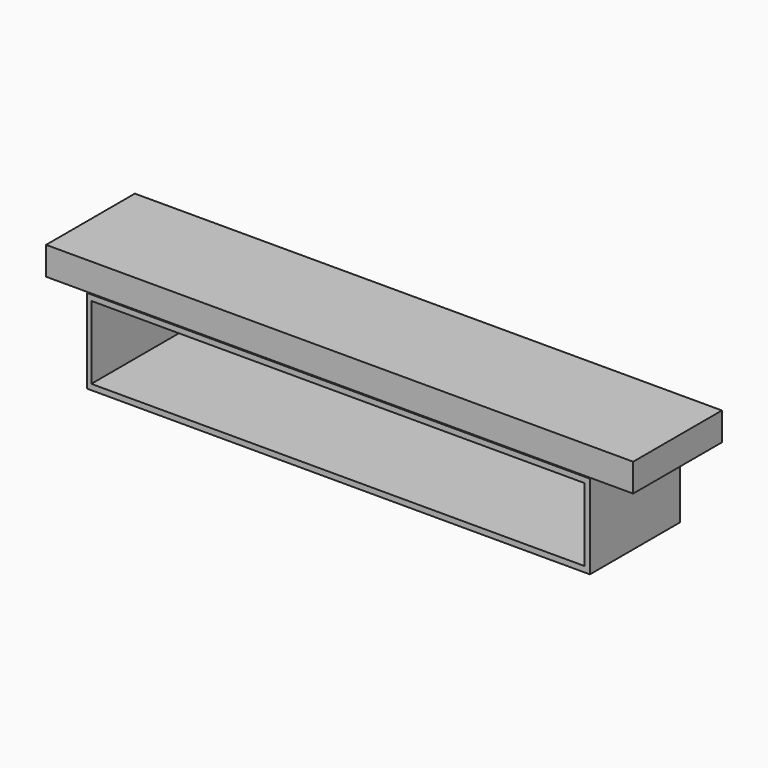
from build123d import *

# Parameters (mm, degrees)
F0_W     = 20
F0_H     = 20
F0_H_2   = 260
F0_W_2   = 15
F0_W_3   = 880
F1_DEPTH = 400
F2_DEPTH = 395


# Not quite as in the source:
# - a feature names something its author has since deleted; it is built from what else it names


with BuildPart() as f1:
    # F0 (on Front) → F1 (new body)
    with BuildSketch(Plane.XZ):
        with Locations((885, -60)):
            Rectangle(F0_W, F0_H)
        Polygon((875, -70), (875, -50), (-5, -50), (-5, -70), (145, -70), align=None)
        with Locations((885, -200)):
            Rectangle(F0_W, F0_H_2)
        Polygon((-5, -70), (-5, -50), (-880, -50), (-880, -70), (-145, -70), align=None)
        with Locations((885, -340)):
            Rectangle(F0_W, F0_H)
        with Locations((-887.5, -60)):
            Rectangle(F0_W_2, F0_H)
        with Locations((435, -340)):
            Rectangle(F0_W_3, F0_H)
        with Locations((-887.5, -200)):
            Rectangle(F0_W_2, F0_H_2)
        Polygon((-5, -350), (-5, -330), (-145, -330), (-880, -330), (-880, -350), (-145, -350), align=None)
        with Locations((-887.5, -340)):
            Rectangle(F0_W_2, F0_H)
    extrude(amount=F1_DEPTH)

    # F0 (on Front) → F2 (join)
    with BuildSketch(Plane.XZ):
        Polygon((895, -50), (1045, -50), (1045, 50), (-1045, 50), (-1045, -50), (-895, -50), (-880, -50), (-5, -50), (875, -50), align=None)
    extrude(amount=F2_DEPTH)


solid = f1.part
